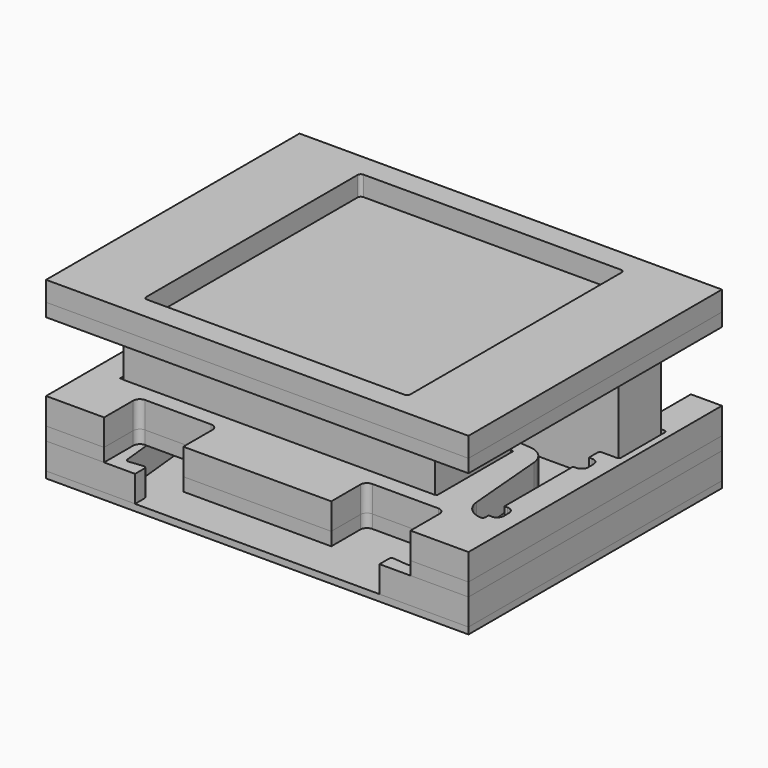
from build123d import *

# Parameters (mm, degrees)
F0_W      = 812.8
F0_H      = 609.6
F1_DEPTH  = 12.7
F3_DEPTH  = 50.8
F5_W      = 812.8
F5_H      = 609.6
F6_DEPTH  = 25.4
F7_W      = 152.4
F7_H      = 82.7492105986
F7_H_2    = 85.014539755
F8_DEPTH  = 25.4
F9_W      = 609.6
F9_H      = 184.15
F10_DEPTH = 50.8
F12_W     = 812.8
F12_H     = 609.6
F13_DEPTH = 25.4
F14_W     = 812.8
F14_H     = 609.6
F14_W_2   = 508
F14_H_2   = 520.7
F15_DEPTH = 38.1
F16_R     = 38.1
F17_R     = 5.08
F18_W     = 774.7
F18_H     = 101.6
F19_DEPTH = 184.15
F18_W_2   = 599.2368
F18_H_2   = 183.2102
F20_R     = 6.35
F21_R     = 12.7
F21_2_R   = 12.7
F22_R     = 5.08
F22_2_R   = 5.08


# Not quite as in the source:
# - a feature names something its author has since deleted; it is built from what else it names


with BuildPart() as f1:
    # F0 (on Top) → F1 (new body)
    with BuildSketch(Plane.XY):
        Rectangle(F0_W, F0_H)
    extrude(amount=F1_DEPTH)


with BuildPart() as f3:
    # F2 (on face) → F3 (new body)
    with BuildSketch(Plane.XY.offset(12.7)):
        Polygon((-292.2997812765, 279.4), (-292.2997812765, 304.8), (-406.4, 304.8), (-406.4, -304.8), (-235.1497812765, -304.8), (-235.1497812765, -276.469874611), (-273.05, -280.36646552), (-330.2, 275.5034090909), align=None)
    extrude(amount=F3_DEPTH)

    # F22
    f22_edges = [f3.edges().sort_by_distance(p)[0] for p in [
        (-330.2, 275.503409, 38.1),
        (-292.299781, 279.4, 38.1),
        (-273.05, -280.366466, 38.1),
        (-235.149781, -276.469875, 38.1),
    ]]
    fillet(f22_edges, radius=F22_R)


with BuildPart() as f3b:
    # F2 (on face) → F3, piece 2 (new body)
    with BuildSketch(Plane.XY.offset(12.7)):
        Polygon((406.4, 304.8), (292.2997812765, 304.8), (292.2997812765, 279.4), (330.2, 275.5034090909), (273.05, -280.36646552), (235.1497812765, -276.469874611), (235.1497812765, -304.8), (406.4, -304.8), align=None)
    extrude(amount=F3_DEPTH)

    # F22#2
    f22_2_edges = [f3b.edges().sort_by_distance(p)[0] for p in [
        (330.2, 275.503409, 38.1),
        (292.299781, 279.4, 38.1),
        (273.05, -280.366466, 38.1),
        (235.149781, -276.469875, 38.1),
    ]]
    fillet(f22_2_edges, radius=F22_2_R)


with BuildPart() as f6:
    # F5 (on offset) → F6 (new body)
    with BuildSketch(Plane.XY.offset(63.5)):
        Rectangle(F5_W, F5_H)
    extrude(amount=F6_DEPTH)

    # F7 (on face) → F8 (cut)
    with BuildSketch(Plane.XY.offset(88.9)):
        with Locations((-218.5643210316, -263.4253947007)):
            Rectangle(F7_W, F7_H)
        with Locations((218.5643210316, -263.4253947007)):
            Rectangle(F7_W, F7_H)
        with Locations((-270.5188664861, 262.2927301225)):
            Rectangle(F7_W, F7_H_2)
        with Locations((270.5188664861, 262.2927301225)):
            Rectangle(F7_W, F7_H_2)
    extrude(amount=-F8_DEPTH, mode=Mode.SUBTRACT)

    # F21
    f21_edges = [f6.edges().sort_by_distance(p)[0] for p in [
        (-294.764321, -222.050789, 76.2),
        (-142.364321, -222.050789, 76.2),
        (294.764321, -222.050789, 76.2),
        (142.364321, -222.050789, 76.2),
        (346.718866, 219.78546, 76.2),
        (-346.718866, 219.78546, 76.2),
        (-194.318866, 219.78546, 76.2),
        (194.318866, 219.78546, 76.2),
    ]]
    fillet(f21_edges, radius=F21_R)


with BuildPart() as f10:
    # F9 (on face) → F10 (new body)
    with BuildSketch(Plane.XY.offset(88.9)):
        Polygon((-406.4, 304.8), (-406.4, -304.8), (-294.7643210316, -304.8), (-294.7643210316, -222.0507894014), (-142.3643210316, -222.0507894014), (-142.3643210316, -304.8), (142.3643210316, -304.8), (142.3643210316, -222.0507894014), (294.7643210316, -222.0507894014), (294.7643210316, -304.8), (406.4, -304.8), (406.4, 304.8), (346.7188664861, 304.8), (346.7188664861, 219.785460245), (194.3188664861, 219.785460245), (194.3188664861, 304.8), (-194.3188664861, 304.8), (-194.3188664861, 219.785460245), (-346.7188664861, 219.785460245), (-346.7188664861, 304.8), align=None)
        with Locations((-50.8, -98.2257894014)):
            Rectangle(F9_W, F9_H, mode=Mode.SUBTRACT)
        Polygon((-393.7, 73.735460245), (-393.7, 188.035460245), (152.4, 188.035460245), (152.4, 226.135460245), (165.1, 226.135460245), (165.1, 188.035460245), (393.7, 188.035460245), (393.7, 73.735460245), (355.6, 73.735460245), (355.6, 48.335460245), (374.65, 48.335460245), (374.65, 10.235460245), (355.6, 10.235460245), (355.6, -154.864539755), (374.65, -154.864539755), (374.65, -192.964539755), (355.6, -192.964539755), (355.6, -205.664539755), (317.5, -205.664539755), (298.45, 16.585460245), (139.7, 29.285460245), (139.7, 73.735460245), align=None, mode=Mode.SUBTRACT)
    extrude(amount=F10_DEPTH)

    # F16
    f16_edges = [f10.edges().sort_by_distance(p)[0] for p in [
        (139.7, 29.28546, 114.3),
        (298.45, 16.58546, 114.3),
        (317.5, -205.66454, 114.3),
    ]]
    fillet(f16_edges, radius=F16_R)

    # F17
    f17_edges = [f10.edges().sort_by_distance(p)[0] for p in [
        (139.7, 73.73546, 114.3),
        (152.4, 188.03546, 114.3),
        (165.1, 188.03546, 114.3),
        (393.7, 188.03546, 114.3),
        (393.7, 73.73546, 114.3),
        (355.6, 73.73546, 114.3),
        (355.6, -205.66454, 114.3),
        (-393.7, 188.03546, 114.3),
        (-393.7, 73.73546, 114.3),
        (165.1, 226.13546, 114.3),
        (152.4, 226.13546, 114.3),
    ]]
    fillet(f17_edges, radius=F17_R)

    # F21#2
    f21_2_edges = [f10.edges().sort_by_distance(p)[0] for p in [
        (-294.764321, -222.050789, 114.3),
        (-142.364321, -222.050789, 114.3),
        (294.764321, -222.050789, 114.3),
        (142.364321, -222.050789, 114.3),
        (-194.318866, 219.78546, 114.3),
        (194.318866, 219.78546, 114.3),
        (346.718866, 219.78546, 114.3),
        (-346.718866, 219.78546, 114.3),
        (374.65, 48.33546, 114.3),
        (374.65, -154.86454, 114.3),
        (374.65, 10.23546, 114.3),
        (374.65, -192.96454, 114.3),
    ]]
    fillet(f21_2_edges, radius=F21_2_R)


with BuildPart() as f13:
    # F12 (on offset) → F13 (new body)
    with BuildSketch(Plane.XY.offset(273.05)):
        Rectangle(F12_W, F12_H)
    extrude(amount=F13_DEPTH)


with BuildPart() as f15:
    # F14 (on face) → F15 (new body)
    with BuildSketch(Plane.XY.offset(298.45)):
        Rectangle(F14_W, F14_H)
        Rectangle(F14_W_2, F14_H_2, mode=Mode.SUBTRACT)
    extrude(amount=F15_DEPTH)

    # F20
    f20_edges = [f15.edges().sort_by_distance(p)[0] for p in [
        (-254, 260.35, 317.5),
        (254, 260.35, 317.5),
        (-254, -260.35, 317.5),
        (254, -260.35, 317.5),
    ]]
    fillet(f20_edges, radius=F20_R)


with BuildPart() as f19:
    # F18 (on face) → F19 (new body)
    with BuildSketch(Plane.XY.offset(88.9)):
        with Locations((0, 130.885460245)):
            Rectangle(F18_W, F18_H)
    extrude(amount=F19_DEPTH)


with BuildPart() as f19b:
    # F18 (on face) → F19, piece 2 (new body)
    with BuildSketch(Plane.XY.offset(88.9)):
        with Locations((-48.7934, -99.4771093487)):
            Rectangle(F18_W_2, F18_H_2)
    extrude(amount=F19_DEPTH)


solid = Compound([f1.part, f3.part, f3b.part, f6.part, f10.part, f13.part, f15.part, f19.part, f19b.part])
